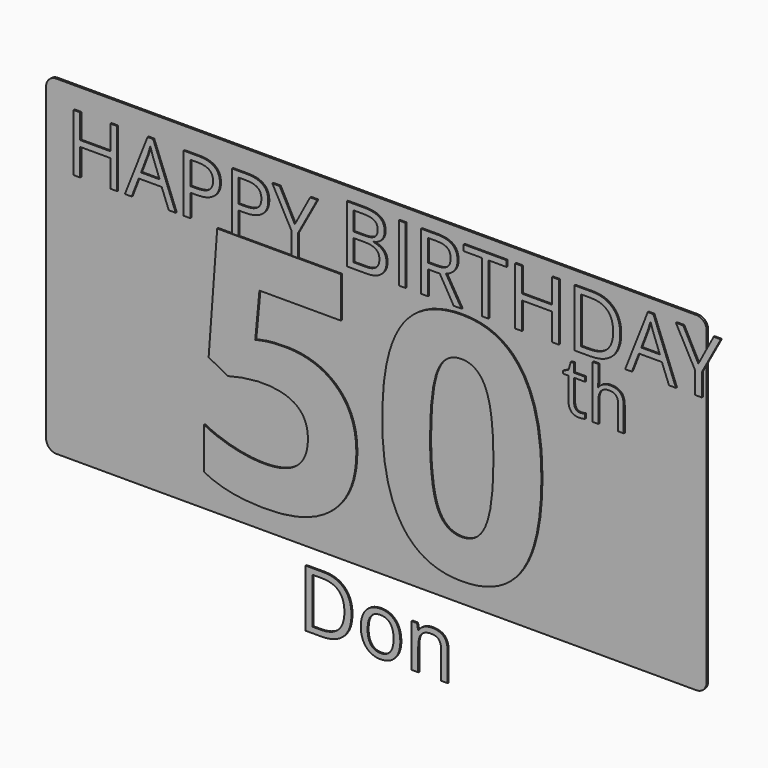
from build123d import *

# Parameters (mm, degrees)
F1_DEPTH       = 0.6
F2_TEXT_SIZE   = 24.6944444444
F2_TEXT_SIZE_2 = 98.1581630916
F2_TEXT_SIZE_3 = 21.381311508
F3_DEPTH       = 0.4


# Not quite as in the source:
# - Text() gives the source's letters only with a copy of the font that has no kerning and outlines rounded to 1/6400 em; it was checked with that copy


with BuildPart() as f1:
    # F0 (on Front) → F1 (new body)
    with BuildSketch(Plane.XZ):
        with BuildLine():
            Line((200.025, 0), (3.175, 0))
            ThreePointArc((3.175, 0), (0.9299359697, -0.9299359697), (0, -3.175))
            Line((0, -3.175), (0, -98.425))
            ThreePointArc((0, -98.425), (0.9299359697, -100.6700640303), (3.175, -101.6))
            Line((3.175, -101.6), (200.025, -101.6))
            ThreePointArc((200.025, -101.6), (202.2700640303, -100.6700640303), (203.2, -98.425))
            Line((203.2, -98.425), (203.2, -3.175))
            ThreePointArc((203.2, -3.175), (202.2700640303, -0.9299359697), (200.025, 0))
        make_face()
    extrude(amount=F1_DEPTH)

    # F2 (on face) → F3 (join)
    with BuildSketch(Plane.XZ.offset(0.6)):
        with Locations((6.35, -24.13)):
            Text('HAPPY', F2_TEXT_SIZE, font='Open Sans', text_align=(TextAlign.LEFT, TextAlign.BOTTOM))
        with Locations((90.4035830206, -21.5067034718)):
            Text('BIRTHDAY', F2_TEXT_SIZE, font='Open Sans', text_align=(TextAlign.LEFT, TextAlign.BOTTOM))
        with Locations((44.139131559, -94.3144559967)):
            Text('50', F2_TEXT_SIZE_2, font='Open Sans', font_style=FontStyle.BOLD, text_align=(TextAlign.LEFT, TextAlign.BOTTOM))
        with Locations((159.060868441, -39.0351228565)):
            Text('th', F2_TEXT_SIZE_3, font='Open Sans', text_align=(TextAlign.LEFT, TextAlign.BOTTOM))
        with Locations((77.7544270833, -124.3073880959)):
            Text('Don', F2_TEXT_SIZE, font='Open Sans', text_align=(TextAlign.LEFT, TextAlign.BOTTOM))
    extrude(amount=F3_DEPTH)


solid = f1.part
